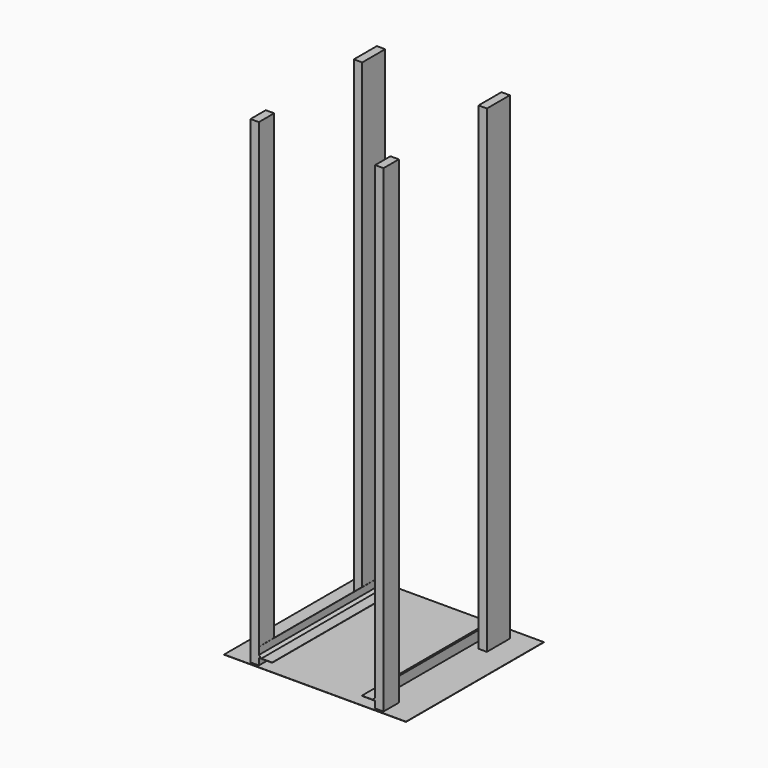
from build123d import *

# Parameters (mm, degrees)
F0_W     = 35
F0_H     = 80
F0_H_2   = 120
F2_DEPTH = 1
F4_DEPTH = 2000
F5_DEPTH = 640


# Not quite as in the source:
# - a feature names something its author has since deleted; it is built from what else it names


with BuildPart() as f2:
    # F0 (on Top) → F2 (new body)
    with BuildSketch(Plane.XY):
        Polygon((380, 360), (-380, 360), (-380, -360), (0, -360), (380, -360), align=None)
        with Locations((-260.5, -310)):
            Rectangle(F0_W, F0_H, mode=Mode.SUBTRACT)
        with Locations((260.5, -310)):
            Rectangle(F0_W, F0_H, mode=Mode.SUBTRACT)
        with Locations((-260.5, 250)):
            Rectangle(F0_W, F0_H_2, mode=Mode.SUBTRACT)
        with Locations((260.5, 250)):
            Rectangle(F0_W, F0_H_2, mode=Mode.SUBTRACT)
    extrude(amount=F2_DEPTH)

    # F0 (on Top) → F4 (join)
    with BuildSketch(Plane.XY):
        with Locations((-260.5, 250)):
            Rectangle(F0_W, F0_H_2)
        with Locations((-260.5, -310)):
            Rectangle(F0_W, F0_H)
        with Locations((260.5, -310)):
            Rectangle(F0_W, F0_H)
        with Locations((260.5, 250)):
            Rectangle(F0_W, F0_H_2)
    extrude(amount=F4_DEPTH)

    # F3 (on offset) → F5 (join)
    with BuildSketch(Plane.XZ.offset(350)):
        Polygon((-187.5, 29), (-187.5, 30), (-232.5, 30), (-242.5, 30), (-242.5, 40), (-242.5, 70), (-243.5, 70), (-243.5, 30), (-243.5, 29), align=None)
        Polygon((-242.5, 30), (-232.5, 30), (-242.5, 40), align=None)
        Polygon((242.5, 40), (232.5, 30), (242.5, 30), align=None)
        Polygon((232.5, 30), (187.5, 30), (187.5, 29), (243.5, 29), (243.5, 30), (243.5, 70), (242.5, 70), (242.5, 40), (242.5, 30), align=None)
    extrude(amount=-F5_DEPTH)


solid = f2.part
